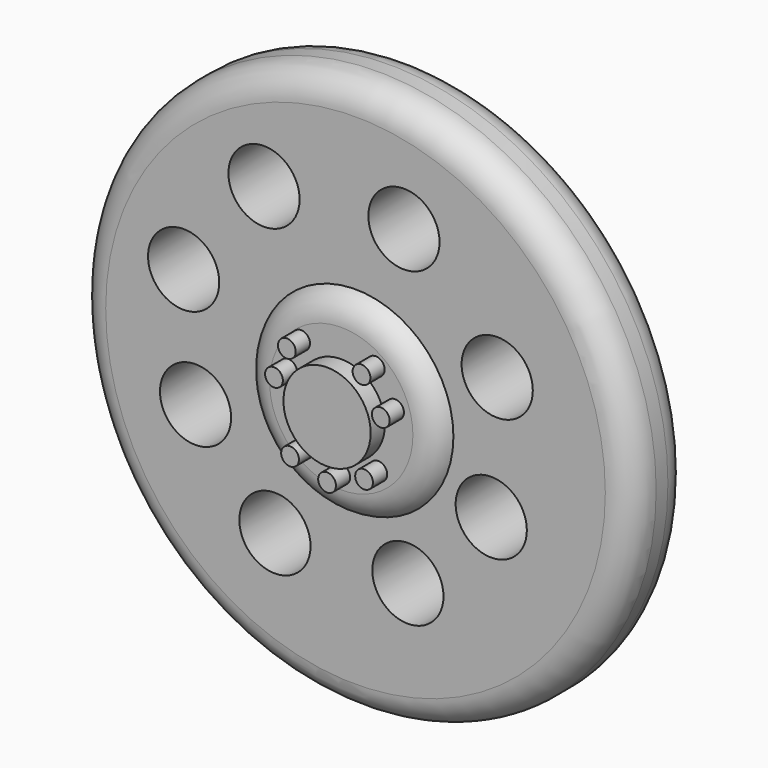
from build123d import *

# Parameters (mm, degrees)
F0_R      = 15.625
F1_DEPTH  = 4
F2_R      = 2.45
F3_DEPTH  = 2
F4_R      = 3
F5_DEPTH  = 9.1
F6_R      = 1.55
F7_DEPTH  = 6
F8_R      = 5.5
F9_DEPTH  = 1
F11_R     = 0.5
F12_DEPTH = 1
F13_R     = 2
F14_DEPTH = 25.4


# Not quite as in the source:
# - a fillet or chamfer that OpenCascade refuses, or shapes differently, is made with other operations: its cross-section is extruded or revolved along the edge and cut away or added


with BuildPart() as f1:
    # F0 (on Front) → F1 (new body)
    with BuildSketch(Plane.XZ):
        Circle(F0_R)
    extrude(amount=F1_DEPTH)

    # F2 (on face) → F3 (join)
    with BuildSketch(Plane.XZ.offset(4)):
        Circle(F2_R)
    extrude(amount=F3_DEPTH)

    # F4 (on face) → F5 (join)
    with BuildSketch(Plane(origin=(0, 0, 0), x_dir=(-1, 0, 0), z_dir=(0, 1, 0))):
        Circle(F4_R)
    extrude(amount=F5_DEPTH)

    # F6 (on face) → F7 (cut)
    with BuildSketch(Plane(origin=(0, 9.1, 0), x_dir=(-1, 0, 0), z_dir=(0, 1, 0))):
        Circle(F6_R)
    extrude(amount=-F7_DEPTH, mode=Mode.SUBTRACT)

    # F8 (on face) → F9 (join)
    with BuildSketch(Plane.XZ.offset(4)):
        Circle(F8_R)
    extrude(amount=F9_DEPTH)

    # F10: fillet of radius 1.5875 on 3 edges, made by hand

    # F10_s1 → F10_t2 (revolve, cut)
    with BuildSketch(Plane.XY):
        with BuildLine():
            ThreePointArc((15.625, -2.4125), (15.1600320151, -3.5350320151), (14.0375, -4))
            Line((14.0375, -4), (15.625, -4))
            Line((15.625, -4), (15.625, -2.4125))
        make_face()
    revolve(axis=Axis((0, -4, 0), (0, -1, 0)), mode=Mode.SUBTRACT)

    # F10_s3 → F10_t4 (revolve, cut)
    with BuildSketch(Plane.XY):
        with BuildLine():
            ThreePointArc((15.625, -1.5875), (15.1600320151, -0.4649679849), (14.0375, 0))
            Line((14.0375, 0), (15.625, 0))
            Line((15.625, 0), (15.625, -1.5875))
        make_face()
    revolve(axis=Axis((0, 0, 0), (0, -1, 0)), mode=Mode.SUBTRACT)

    # F10_s5 → F10_t6 (revolve, cut)
    with BuildSketch(Plane.XY):
        with BuildLine():
            ThreePointArc((5.5, -4), (4.9161383637, -4.7264277948), (4.0252118796, -5))
            Line((4.0252118796, -5), (5.5, -5))
            Line((5.5, -5), (5.5, -4))
        make_face()
    revolve(axis=Axis((0, -5, 0), (0, -1, 0)), mode=Mode.SUBTRACT)

    # F11 (on face) → F12 (join)
    with BuildSketch(Plane.XZ.offset(5)):
        with Locations((-2.9818608891, 0.9871639777)):
            Circle(F11_R)
        with Locations((-2.258730121, 2.6503647678)):
            Circle(F11_R)
        with Locations((1.9354285905, 2.7226777747)):
            Circle(F11_R)
        with Locations((3.0201247428, 0.9510074742)):
            Circle(F11_R)
        with Locations((2.0800547209, -2.4115508422)):
            Circle(F11_R)
        with Locations((0, -3.2431513537)):
            Circle(F11_R)
        with Locations((-2.0779473707, -2.628490096)):
            Circle(F11_R)
    extrude(amount=F12_DEPTH)

    # F13 (on face) → F14 (cut)
    with BuildSketch(Plane.XZ.offset(4)):
        with Locations((-5.1422282122, 8.9166210964)):
            Circle(F13_R)
        with Locations((2.720073564, 9.3627097085)):
            Circle(F13_R)
        with Locations((7.9616084695, 3.7308477331)):
            Circle(F13_R)
        with Locations((7.6270420104, -3.2950392924)):
            Circle(F13_R)
        with Locations((2.9431174044, -8.0904858187)):
            Circle(F13_R)
        with Locations((-4.5288573019, -8.0347247422)):
            Circle(F13_R)
        with Locations((-8.9897383004, -3.1277562957)):
            Circle(F13_R)
        with Locations((-9.6588702872, 3.3405206632)):
            Circle(F13_R)
    extrude(amount=-F14_DEPTH, mode=Mode.SUBTRACT)


solid = f1.part
